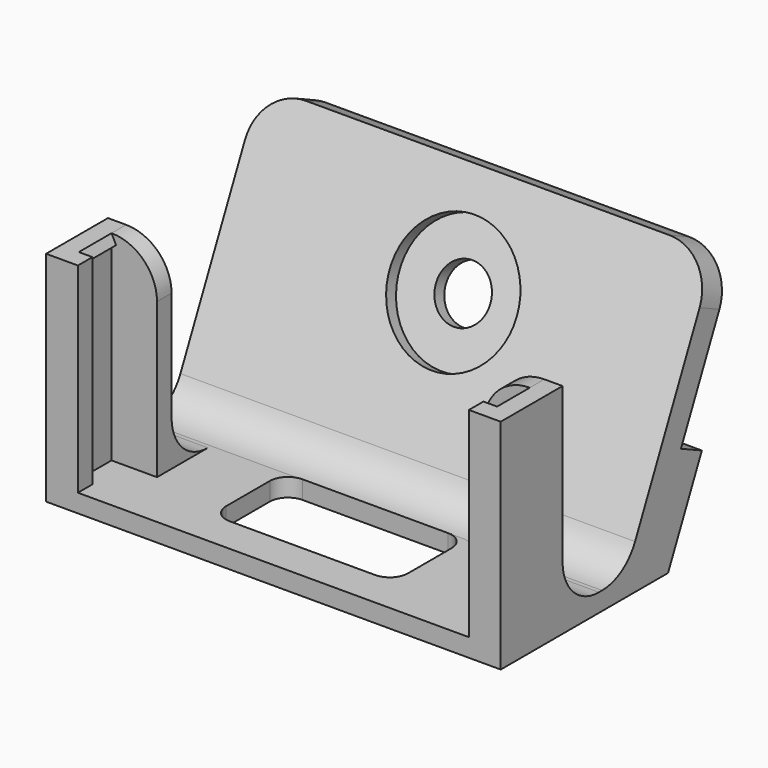
from build123d import *

# Parameters (mm, degrees)
F1_DEPTH      = 50
F3_DEPTH      = 3
F5_DEPTH      = 6.5
F6_W          = 2
F6_H          = 22
F5_FACE1_W    = 6.5
F5_FACE1_H    = 22
F7_DEPTH      = 1.5
F8_W          = 2
F8_H          = 22
F9_DEPTH      = 1.5
F10_W         = 36
F10_H         = 22
F11_DEPTH     = 2
F12_W         = 20
F12_H         = 10
F13_DEPTH     = 28.4580883963
F14_T4_DEPTH  = 50
F14_T10_DEPTH = 50
F14_T16_DEPTH = 50
F14_T23_DEPTH = 50
F14_T29_DEPTH = 50
F15_R         = 5
F16_T4_DEPTH  = 7.0003952761
F17_R         = 2
F18_R         = 2
F19_R         = 7
F19_R_2       = 3
F20_DEPTH     = 1.5
F22_DEPTH     = 4.5
F24_DEPTH     = 4.5
F25_R         = 5
F26_R         = 5


# Not quite as in the source:
# - a fillet or chamfer that OpenCascade refuses, or shapes differently, is made with other operations: its cross-section is extruded or revolved along the edge and cut away or added


with BuildPart() as f1:
    # F0 (on Right) → F1 (new body)
    with BuildSketch(Plane.YZ):
        Polygon((-2, 0), (0, 0), (0, 2), (0, 24), (-2, 24), align=None)
        Polygon((0, 2), (0, 0), (11, 0), (16.274498548, 11.3111986384), (23.6785478522, 27.1892336111), (20.9596244911, 28.4570883963), (8.6224815594, 2), align=None)
        Polygon((16.274498548, 11.3111986384), (11, 0), (14.5032248927, 0), (19.1520257719, 9.9693856574), align=None)
    extrude(amount=F1_DEPTH)

    # F2 (on face) → F3 (cut, through all)
    with BuildSketch(Plane(origin=(0, 6.3164084922, -2.9453896519), x_dir=(1, 0, 0), z_dir=(0, -0.906307787, 0.4226182617))):
        with BuildLine():
            ThreePointArc((22, 23.4566337426), (25, 20.4566337426), (28, 23.4566337426))
            Line((28, 23.4566337426), (22, 23.4566337426))
        make_face()
        with BuildLine():
            Line((22, 23.4566337426), (28, 23.4566337426))
            ThreePointArc((28, 23.4566337426), (25, 26.4566337426), (22, 23.4566337426))
        make_face()
    extrude(amount=-F3_DEPTH, mode=Mode.SUBTRACT)

    # F4 (on face) → F5 (join)
    with BuildSketch(Plane.XZ.offset(2)):
        Polygon((2, 2), (2, 24), (0, 24), (0, 0), (50, 0), (50, 24), (48, 24), (48, 2), align=None)
    extrude(amount=F5_DEPTH)

    # F6 (on face) + F5_face1 (on face) → F7 (join)
    with BuildSketch(Plane.YZ.offset(2)):
        with Locations((-7.5, 13)):
            Rectangle(F6_W, F6_H)
    with BuildSketch(Plane(origin=(48, -5.25, 13), x_dir=(0, -1, 0), z_dir=(-1, 0, 0))):
        Rectangle(F5_FACE1_W, F5_FACE1_H)
    extrude(amount=F7_DEPTH, dir=(1, 0, 0))

    # F8 (on face) → F9 (join)
    with BuildSketch(Plane(origin=(48, 0, 0), x_dir=(0, -1, 0), z_dir=(-1, 0, 0))):
        with Locations((7.5, 13)):
            Rectangle(F8_W, F8_H)
    extrude(amount=F9_DEPTH)

    # F10 (on face) → F11 (cut)
    with BuildSketch(Plane.XZ.offset(2)):
        with Locations((25, 13)):
            Rectangle(F10_W, F10_H)
    extrude(amount=-F11_DEPTH, mode=Mode.SUBTRACT)

    # F12 (on Top) → F13 (cut, through all)
    with BuildSketch(Plane.XY):
        with Locations((25, 0.5)):
            Rectangle(F12_W, F12_H)
    extrude(amount=F13_DEPTH, mode=Mode.SUBTRACT)

    # F14: fillet of radius 5 on 1 edges, made by hand


with BuildPart() as f14_tool2:
    # F14_s3 → F14_t4 (new body)
    with BuildSketch(Plane.YZ):
        with BuildLine():
            ThreePointArc((9.9686691906, 4.8869086913), (8.1236282971, 2.7830427709), (5.4371302554, 2))
            Line((5.4371302554, 2), (8.6224815594, 2))
            Line((8.6224815594, 2), (9.9686691906, 4.8869086913))
        make_face()
    extrude(amount=F14_T4_DEPTH)

    split(bisect_by=Plane.XZ.offset(-5.5), keep=Keep.BOTTOM)

    split(bisect_by=Plane.YZ.offset(15), keep=Keep.BOTTOM)


with BuildPart() as f1_1:
    add(f1.part)

    # F14_t1: union F14_tool2
    add(f14_tool2.part)


with BuildPart() as f14_tool8:
    # F14_s9 → F14_t10 (new body)
    with BuildSketch(Plane.YZ):
        with BuildLine():
            ThreePointArc((9.9686691906, 4.8869086913), (8.1236282971, 2.7830427709), (5.4371302554, 2))
            Line((5.4371302554, 2), (8.6224815594, 2))
            Line((8.6224815594, 2), (9.9686691906, 4.8869086913))
        make_face()
    extrude(amount=F14_T10_DEPTH)

    split(bisect_by=Plane.XZ.offset(-5.5), keep=Keep.TOP)

    split(bisect_by=Plane.YZ.offset(15), keep=Keep.BOTTOM)


with BuildPart() as f1_2:
    add(f1_1.part)

    # F14_t7: union F14_tool8
    add(f14_tool8.part)


with BuildPart() as f14_tool14:
    # F14_s15 → F14_t16 (new body)
    with BuildSketch(Plane.YZ):
        with BuildLine():
            ThreePointArc((9.9686691906, 4.8869086913), (8.1236282971, 2.7830427709), (5.4371302554, 2))
            Line((5.4371302554, 2), (8.6224815594, 2))
            Line((8.6224815594, 2), (9.9686691906, 4.8869086913))
        make_face()
    extrude(amount=F14_T16_DEPTH)

    split(bisect_by=Plane.XZ.offset(-5.5), keep=Keep.BOTTOM)

    split(bisect_by=Plane.YZ.offset(15), keep=Keep.TOP)

    split(bisect_by=Plane.YZ.offset(35), keep=Keep.BOTTOM)


with BuildPart() as f1_3:
    add(f1_2.part)

    # F14_t13: union F14_tool14
    add(f14_tool14.part)


with BuildPart() as f14_tool21:
    # F14_s22 → F14_t23 (new body)
    with BuildSketch(Plane.YZ):
        with BuildLine():
            ThreePointArc((9.9686691906, 4.8869086913), (8.1236282971, 2.7830427709), (5.4371302554, 2))
            Line((5.4371302554, 2), (8.6224815594, 2))
            Line((8.6224815594, 2), (9.9686691906, 4.8869086913))
        make_face()
    extrude(amount=F14_T23_DEPTH)

    split(bisect_by=Plane.XZ.offset(-5.5), keep=Keep.BOTTOM)

    split(bisect_by=Plane.YZ.offset(35), keep=Keep.TOP)


with BuildPart() as f1_4:
    add(f1_3.part)

    # F14_t20: union F14_tool21
    add(f14_tool21.part)


with BuildPart() as f14_tool27:
    # F14_s28 → F14_t29 (new body)
    with BuildSketch(Plane.YZ):
        with BuildLine():
            ThreePointArc((9.9686691906, 4.8869086913), (8.1236282971, 2.7830427709), (5.4371302554, 2))
            Line((5.4371302554, 2), (8.6224815594, 2))
            Line((8.6224815594, 2), (9.9686691906, 4.8869086913))
        make_face()
    extrude(amount=F14_T29_DEPTH)

    split(bisect_by=Plane.XZ.offset(-5.5), keep=Keep.TOP)

    split(bisect_by=Plane.YZ.offset(35), keep=Keep.TOP)


with BuildPart() as f1_5:
    add(f1_4.part)

    # F14_t26: union F14_tool27
    add(f14_tool27.part)

    # F15
    f15_edges = [f1_5.edges().sort_by_distance(p)[0] for p in [
        (3.5, 0, 2),
        (46.5, 0, 2),
    ]]
    fillet(f15_edges, radius=F15_R)

    # F16: fillet of radius 2 on 1 edges, made by hand


with BuildPart() as f16_tool2:
    # F16_s3 → F16_t4 (new body)
    with BuildSketch(Plane.XY):
        with BuildLine():
            ThreePointArc((35, 3.5), (34.4142135624, 4.9142135624), (33, 5.5))
            Line((33, 5.5), (33, 5.54))
            Line((33, 5.54), (35.04, 5.54))
            Line((35.04, 5.54), (35.04, 3.5))
            Line((35.04, 3.5), (35, 3.5))
        make_face()
    extrude(amount=F16_T4_DEPTH)

    split(bisect_by=Plane.XY.offset(2), keep=Keep.BOTTOM)


with BuildPart() as f1_6:
    add(f1_5.part)

    # F16_t1: union F16_tool2
    add(f16_tool2.part)

    # F17#2 (call 1 of 2: OpenCascade refuses the feature's edges together)
    f17_2_edges = [f1_6.edges().sort_by_distance(p)[0] for p in [
        (15, -4.5, 1),
    ]]
    fillet(f17_2_edges, radius=F17_R)

    # F17 (call 2 of 2)
    f17_edges = [f1_6.edges().sort_by_distance(p)[0] for p in [
        (15, 5.5, 1.000198),
    ]]
    fillet(f17_edges, radius=F17_R)

    # F18
    f18_edges = [f1_6.edges().sort_by_distance(p)[0] for p in [
        (35, -4.5, 1),
    ]]
    fillet(f18_edges, radius=F18_R)

    # F19 (on face) → F20 (cut)
    with BuildSketch(Plane(origin=(0, 6.3164084922, -2.9453896519), x_dir=(1, 0, 0), z_dir=(0, -0.906307787, 0.4226182617))):
        with Locations((25, 23.4566337426)):
            Circle(F19_R)
        with Locations((25, 23.4566337426)):
            Circle(F19_R_2, mode=Mode.SUBTRACT)
    extrude(amount=-F20_DEPTH, mode=Mode.SUBTRACT)

    # F21 (on face) → F22 (join, through all)
    with BuildSketch(Plane.XZ.offset(2)):
        Polygon((48, 23), (48, 24), (47.5, 23), align=None)
    extrude(amount=F22_DEPTH)

    # F23 (on face) → F24 (join, through all)
    with BuildSketch(Plane.XZ.offset(2)):
        Polygon((2.5, 23), (2, 24), (2, 23), align=None)
    extrude(amount=F24_DEPTH)

    # F25
    f25_edges = [f1_6.edges().sort_by_distance(p)[0] for p in [
        (50, 22.319086, 27.823161),
        (0, 22.319086, 27.823161),
    ]]
    fillet(f25_edges, radius=F25_R)

    # F26
    f26_edges = [f1_6.edges().sort_by_distance(p)[0] for p in [
        (7, -1, 24),
        (43, -1, 24),
    ]]
    fillet(f26_edges, radius=F26_R)


solid = f1_6.part
